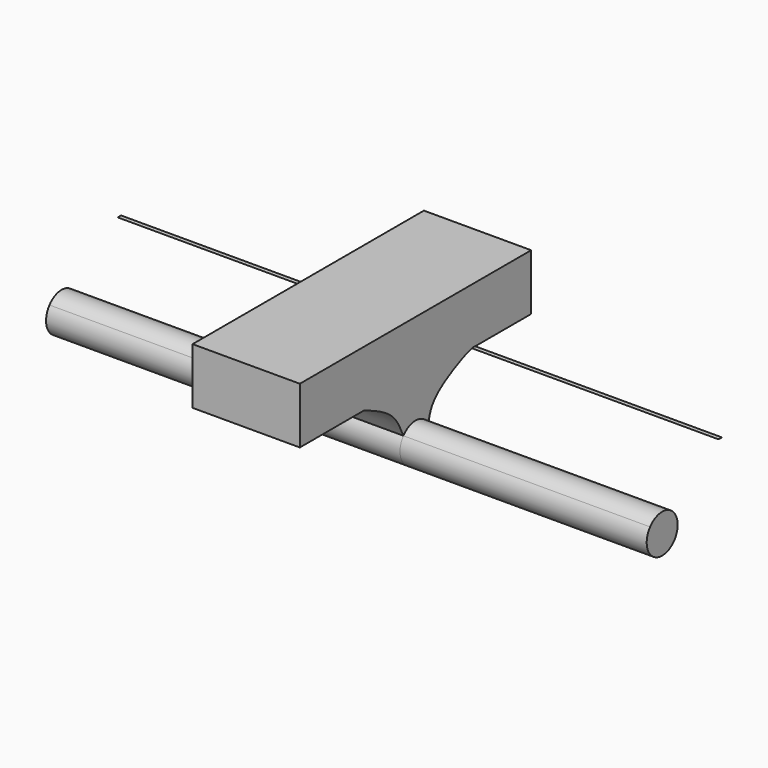
from build123d import *

# Parameters (mm, degrees)
F1_DEPTH = 71.12
F2_DEPTH = 12.7


with BuildPart() as f1:
    # F0 (on Right) → F1 (new body, symmetric)
    with BuildSketch(Plane.YZ):
        with BuildLine():
            ThreePointArc((-3.5772807297, -10.0167868583), (-1.5196570548, -17.2098026647), (4.5847, -12.8842834444))
            ThreePointArc((4.5847, -12.8842834444), (4.3928679628, -11.5719629228), (3.8334250414, -10.3694620706))
            ThreePointArc((3.8334250414, -10.3694620706), (0.2179390476, -8.304766367), (-3.5772807297, -10.0167868583))
        make_face()
    extrude(amount=F1_DEPTH, both=True)


with BuildPart() as f1b:
    # F0 (on Right) → F1, piece 2 (new body, symmetric)
    with BuildSketch(Plane.YZ):
        with BuildLine():
            add(Edge.make_bspline(
                [(16.6792012751, 0), (17.2352067537, 0.12198039), (17.4606638005, 0.0610249655), (17.682461068, 0)],
                knots=[0.8521618943, 0.8521618943, 0.8521618943, 0.8521618943, 1, 1, 1, 1], degree=3))
            Line((16.6792012751, 0), (17.682461068, 0))
        make_face()
    extrude(amount=F1_DEPTH, both=True)


with BuildPart() as f2:
    # F0 (on Right) → F2 (new body, symmetric)
    with BuildSketch(Plane.YZ):
        with BuildLine():
            ThreePointArc((-3.5772807297, -10.0167868583), (-1.5196570548, -17.2098026647), (4.5847, -12.8842834444))
            ThreePointArc((4.5847, -12.8842834444), (4.3928679628, -11.5719629228), (3.8334250414, -10.3694620706))
            ThreePointArc((3.8334250414, -10.3694620706), (0.2179390476, -8.304766367), (-3.5772807297, -10.0167868583))
        make_face()
        with BuildLine():
            ThreePointArc((-3.5772807297, -10.0167868583), (0.2179390476, -8.304766367), (3.8334250414, -10.3694620706))
            add(Edge.make_bspline(
                [(3.8334250414, -10.3694620706), (4.1484940345, -8.7462774015), (5.1007491044, -4.7054371148), (14.7876531546, -0.4149811222), (16.6792012751, 0)],
                knots=[0, 0, 0, 0, 0.3492120103, 0.8521618943, 0.8521618943, 0.8521618943, 0.8521618943], degree=3))
            Line((16.6792012751, 0), (-15.1743106544, 0))
            add(Edge.make_bspline(
                [(-3.5772807297, -10.0167868583), (-4.4214296894, -8.1091133852), (-6.3202305252, -3.8500304601), (-12.0298605248, -1.3672692408), (-15.1743106544, 0)],
                knots=[0, 0, 0, 0, 0.4493592658, 1, 1, 1, 1], degree=3))
        make_face()
        with BuildLine():
            Line((-15.1743106544, 0), (16.6792012751, 0))
            add(Edge.make_bspline(
                [(16.6792012751, 0), (17.2352067537, 0.12198039), (17.4606638005, 0.0610249655), (17.682461068, 0)],
                knots=[0.8521618943, 0.8521618943, 0.8521618943, 0.8521618943, 1, 1, 1, 1], degree=3))
            Line((17.682461068, 0), (34.2362560332, 0))
            Line((34.2362560332, 0), (34.2362560332, 13.2931983098))
            Line((34.2362560332, 13.2931983098), (-34.2362560332, 13.2931983098))
            Line((-34.2362560332, 13.2931983098), (-34.2362560332, 0))
            Line((-34.2362560332, 0), (-15.1743106544, 0))
        make_face()
        with BuildLine():
            add(Edge.make_bspline(
                [(16.6792012751, 0), (17.2352067537, 0.12198039), (17.4606638005, 0.0610249655), (17.682461068, 0)],
                knots=[0.8521618943, 0.8521618943, 0.8521618943, 0.8521618943, 1, 1, 1, 1], degree=3))
            Line((16.6792012751, 0), (17.682461068, 0))
        make_face()
    extrude(amount=F2_DEPTH, both=True)


solid = Compound([f1.part, f1b.part, f2.part])
